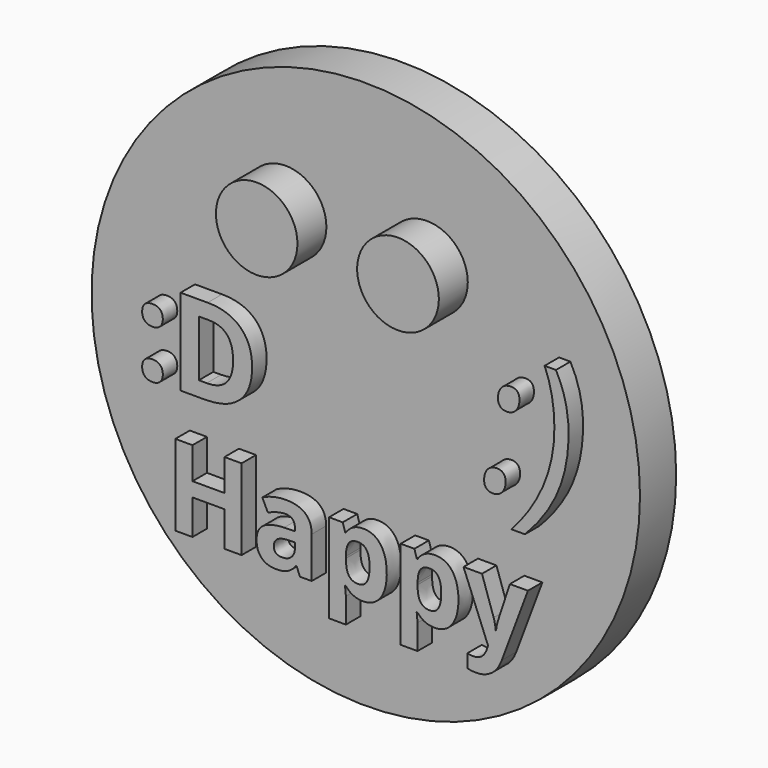
from build123d import *

# Parameters (mm, degrees)
F0_R         = 30.3302860692
F1_DEPTH     = 5
F2_R         = 4.5185950883
F2_R_2       = 4.5085884631
F3_DEPTH     = 9
F4_TEXT_SIZE = 12.5238581354
F5_DEPTH     = 7
F6_TEXT_SIZE = 19.6207068964
F7_DEPTH     = 7
F8_TEXT_SIZE = 13.358779769
F9_DEPTH     = 7


# Not quite as in the source:
# - Text() gives the source's letters only with a copy of the font that has no kerning and outlines rounded to 1/6400 em; it was checked with that copy


with BuildPart() as f1:
    # F0 (on Front) → F1 (new body)
    with BuildSketch(Plane.XZ):
        Circle(F0_R)
    extrude(amount=F1_DEPTH)

    # F2 (on Front) → F3 (join)
    with BuildSketch(Plane.XZ):
        with Locations((6.7628822289, 14.5777678117)):
            Circle(F2_R)
        with Locations((-8.8668903336, 14.8783409968)):
            Circle(F2_R_2)
    extrude(amount=F3_DEPTH)

    # F4 (on Front) → F5 (join)
    with BuildSketch(Plane.XZ):
        with Locations((-20.5892185622, -18.7857849523)):
            Text('Happy', F4_TEXT_SIZE, font='Open Sans', font_style=FontStyle.BOLD, text_align=(TextAlign.LEFT, TextAlign.BOTTOM))
    extrude(amount=F5_DEPTH)

    # F6 (on Front) → F7 (join)
    with BuildSketch(Plane.XZ):
        with Locations((14.2771946266, -3.4565837122)):
            Text(':)', F6_TEXT_SIZE, font='Open Sans', font_style=FontStyle.ITALIC, text_align=(TextAlign.LEFT, TextAlign.BOTTOM))
    extrude(amount=F7_DEPTH)

    # F8 (on Front) → F9 (join)
    with BuildSketch(Plane.XZ):
        with Locations((-23.8955169916, -4.9594468437)):
            Text(':D', F8_TEXT_SIZE, font='Open Sans', font_style=FontStyle.BOLD, text_align=(TextAlign.LEFT, TextAlign.BOTTOM))
    extrude(amount=F9_DEPTH)


solid = f1.part
